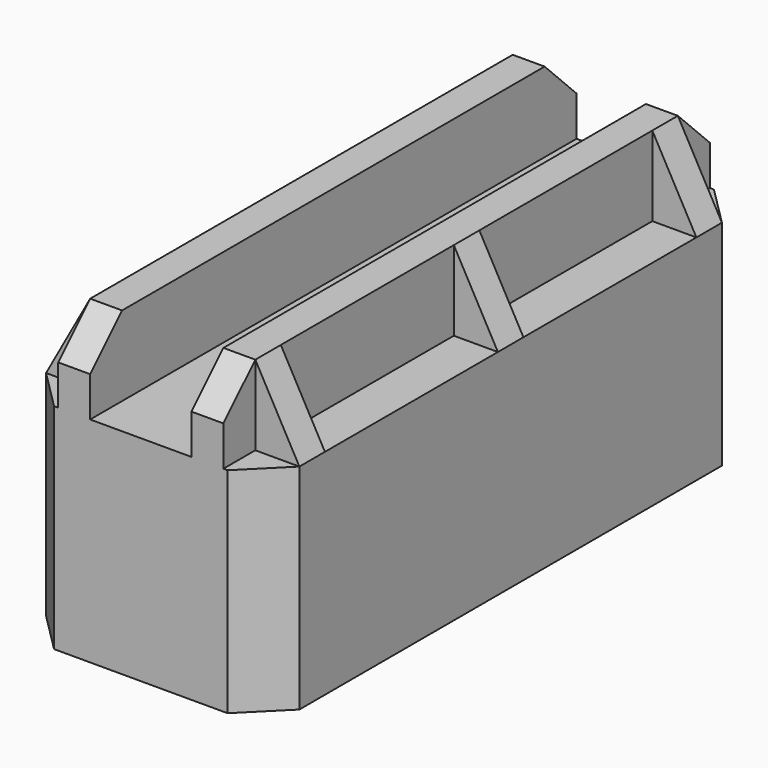
from build123d import *

# Parameters (mm, degrees)
F0_W      = 31.75
F0_H      = 76.2
F1_DEPTH  = 26.81
F2_SIZE   = 5
F3_T      = -4
F4_W      = 4
F4_H      = 10
F5_DEPTH  = 38.1
F7_DEPTH  = 2
F10_DEPTH = 4
F11_SIZE  = 5


# Not quite as in the source:
# - a pattern or mirror of a feature is missing from the dataset's text; its kind, count and spacing are read off the source's solid


with BuildPart() as f1:
    # F0 (on Top) → F1 (new body)
    with BuildSketch(Plane.XY):
        Rectangle(F0_W, F0_H)
    extrude(amount=-F1_DEPTH)

    # F2
    f2_edges = [f1.edges().sort_by_distance(p)[0] for p in [
        (-15.875, -38.1, -13.405),
        (15.875, -38.1, -13.405),
        (-15.875, 38.1, -13.405),
        (15.875, 38.1, -13.405),
    ]]
    chamfer(f2_edges, length=F2_SIZE)

    # F3
    f3_openings = [f1.faces().sort_by_distance(p)[0] for p in [
        (0, 0, -26.81),
    ]]
    offset(amount=F3_T, openings=f3_openings)

    # F4 (on Front) → F5 (join, symmetric)
    with BuildSketch(Plane.XZ):
        with Locations((8.35, 5)):
            Rectangle(F4_W, F4_H)
        with Locations((-8.35, 5)):
            Rectangle(F4_W, F4_H)
    extrude(amount=F5_DEPTH, both=True)

    # F6 (on Front) → F7 (join, symmetric)
    with BuildSketch(Plane.XZ):
        Polygon((-15.875, 0), (-10.35, 0), (-10.35, 10), align=None)
        Polygon((15.875, 0), (10.35, 10), (10.35, 0), align=None)
    f7 = extrude(amount=F7_DEPTH, both=True)

    # F7_copies: F7 across plane
    add(f7.mirror(Plane.ZX.offset(15.55)))

    # F9 (on face) → F10 (join)
    with BuildSketch(Plane.XZ.offset(33.1)):
        Polygon((-10.35, 0), (-10.35, 10), (-15.875, 0), align=None)
        Polygon((10.35, 10), (10.35, 0), (15.875, 0), align=None)
    extrude(amount=-F10_DEPTH)

    # F11
    f11_edges = [f1.edges().sort_by_distance(p)[0] for p in [
        (-8.35, -38.1, 10),
        (8.35, -38.1, 10),
        (-8.35, 38.1, 10),
        (8.35, 38.1, 10),
    ]]
    chamfer(f11_edges, length=F11_SIZE)


solid = f1.part
